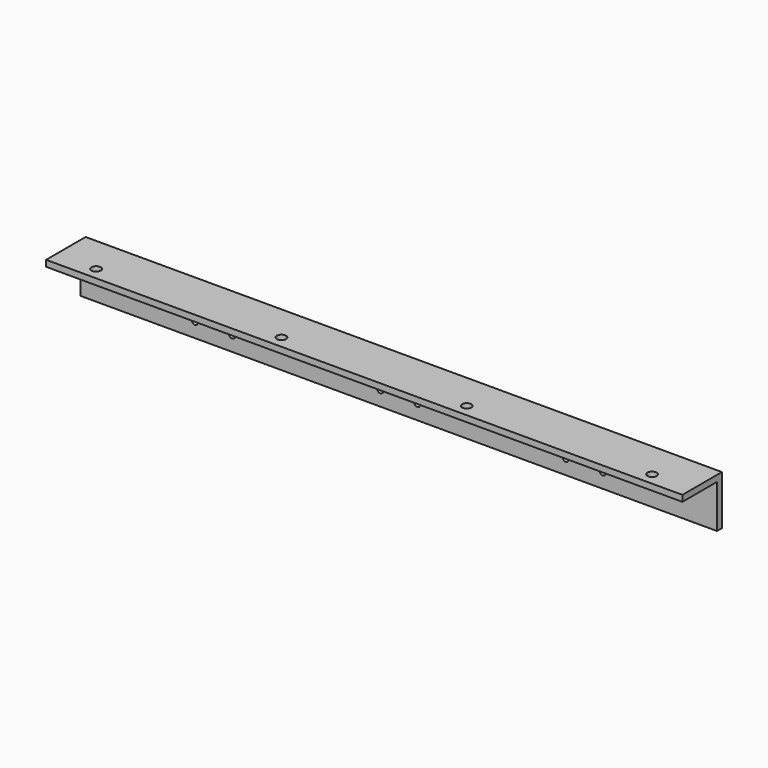
from build123d import *

# Parameters (mm, degrees)
F1_DEPTH      = 327.025
F2_R          = 4.7625
F3_DEPTH      = 50.801
F4_R          = 3.175
F5_DEPTH      = 50.801
F5_DEPTH_BACK = 697


# Not quite as in the source:
# - an extrude ends at something that could not be found from the text; its depth is read off the source's solid


with BuildPart() as f1:
    # F0 (on Right) → F1 (new body, symmetric)
    with BuildSketch(Plane.YZ):
        Polygon((0, 44.45), (0, 0), (6.35, 0), (6.35, 50.8), (-44.45, 50.8), (-44.45, 44.45), align=None)
    extrude(amount=F1_DEPTH, both=True)

    # F2 (on face) → F3 (cut, through all)
    with BuildSketch(Plane.XY.offset(50.8)):
        with Locations((-285.75, -31.75)):
            Circle(F2_R)
        with Locations((-95.25, -31.75)):
            Circle(F2_R)
        with Locations((95.25, -31.75)):
            Circle(F2_R)
        with Locations((285.75, -31.75)):
            Circle(F2_R)
    extrude(amount=-F3_DEPTH, mode=Mode.SUBTRACT)

    # F4 (on face) → F5 (cut, two sides)
    with BuildSketch(Plane(origin=(0, 6.35, 0), x_dir=(-1, 0, 0), z_dir=(0, 1, 0))) as f5_sk:
        with Locations((209.55, 15.24)):
            Circle(F4_R)
        with Locations((171.45, 15.24)):
            Circle(F4_R)
        with Locations((19.05, 15.24)):
            Circle(F4_R)
        with Locations((-19.05, 15.24)):
            Circle(F4_R)
        with Locations((-171.45, 15.24)):
            Circle(F4_R)
        with Locations((-209.55, 15.24)):
            Circle(F4_R)
    extrude(amount=-F5_DEPTH, mode=Mode.SUBTRACT)
    extrude(f5_sk.sketch, amount=F5_DEPTH_BACK, mode=Mode.SUBTRACT)


solid = f1.part
